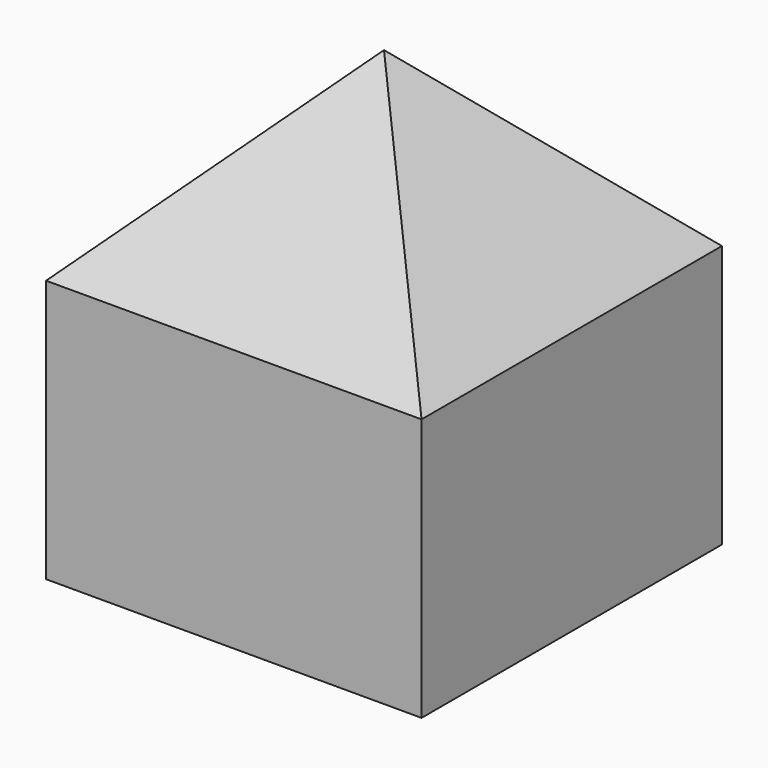
from build123d import *

# Parameters (mm, degrees)
F0_R     = 381
F1_DEPTH = 762
F3_W     = 50
F3_H     = 50
F3_W_2   = 40
F3_H_2   = 40
F4_DEPTH = 30
F5_W     = 50
F5_H     = 50
F5_W_2   = 40
F5_H_2   = 40
F6_DEPTH = 30
F7_SIZE  = 24.99999


# Not quite as in the source:
# - a fillet or chamfer is up to 0.001 mm smaller than in the source, because OpenCascade refuses the exact size


with BuildPart() as f1:
    # F0 (on Top) → F1 (new body)
    with BuildSketch(Plane.XY):
        Circle(F0_R)
    extrude(amount=F1_DEPTH)


with BuildPart() as f4:
    # F3 (on Top) → F4 (new body)
    with BuildSketch(Plane.XY):
        Rectangle(F3_W, F3_H)
        Rectangle(F3_W_2, F3_H_2, mode=Mode.SUBTRACT)
    extrude(amount=F4_DEPTH)

    # F5 (on face) → F6 (join)
    with BuildSketch(Plane.XY.offset(30)):
        Rectangle(F5_W, F5_H)
        Rectangle(F5_W_2, F5_H_2, mode=Mode.SUBTRACT)
        Rectangle(F5_W_2, F5_H_2)
    extrude(amount=F6_DEPTH)

    # F7 (size 25 in the source; OpenCascade refuses exactly that, so slightly less here)
    f7_edges = [f4.edges().sort_by_distance(p)[0] for p in [
        (25, 0, 60),
        (0, 25, 60),
        (-25, 0, 60),
        (0, -25, 60),
    ]]
    chamfer(f7_edges, length=F7_SIZE)


solid = f4.part
